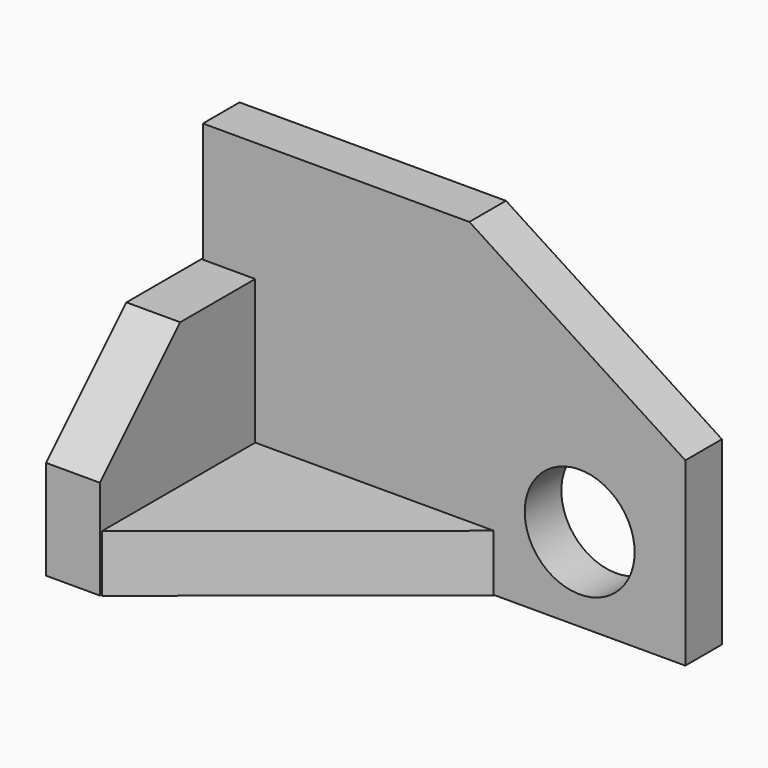
from build123d import *

# Parameters (mm, degrees)
F0_R      = 12.5067254218
F1_DEPTH  = 10.414
F2_W      = 12.2419670224
F2_H      = 45.4701641575
F3_DEPTH  = 54.61
F4_SIZE   = 22.86
F6_DEPTH  = 30.734
F8_DEPTH  = 17.78
F9_W      = 56.2547529116
F9_H      = 22.1521309577
F10_DEPTH = 10.414


# Not quite as in the source:
# - a feature names something its author has since deleted; it is built from what else it names


with BuildPart() as f1:
    # F0 (on Front) → F1 (new body)
    with BuildSketch(Plane.XZ):
        Polygon((5.0146179641, 42.2928149286), (-55.6240000051, 42.2928149286), (-55.6240000051, -30.6337999585), (54.1666180116, -30.6337999585), (54.1666180116, 10.5042919132), align=None)
        with Locations((30.1248802542, -11.6675363407)):
            Circle(F0_R, mode=Mode.SUBTRACT)
    extrude(amount=F1_DEPTH)

    # F2 (on Front) → F3 (join)
    with BuildSketch(Plane.XZ):
        with Locations((-49.8422943056, -7.7240983956)):
            Rectangle(F2_W, F2_H)
    extrude(amount=F3_DEPTH)

    # F4
    f4_edges = [f1.edges().sort_by_distance(p)[0] for p in [
        (-49.842294, -54.61, 15.010984),
    ]]
    chamfer(f4_edges, length=F4_SIZE)

    # F5 (on Top) → F6 (join)
    with BuildSketch(Plane.XY):
        Polygon((11.3675408065, -9.7644263878), (-43.7213107944, -9.7644263878), (-43.7213107944, -54.0686920285), align=None)
    extrude(amount=-F6_DEPTH)

    # F7 (on Top) → F8 (cut)
    with BuildSketch(Plane.XY):
        Polygon((11.3675408065, -10.3473765776), (-43.7213107944, -10.3473765776), (-43.7213107944, -55.2345886827), align=None)
    extrude(amount=-F8_DEPTH, mode=Mode.SUBTRACT)

    # F9 (on Front) → F10 (join)
    with BuildSketch(Plane.XZ):
        with Locations((-15.5939343385, -6.8496719468)):
            Rectangle(F9_W, F9_H)
    extrude(amount=F10_DEPTH)


solid = f1.part
